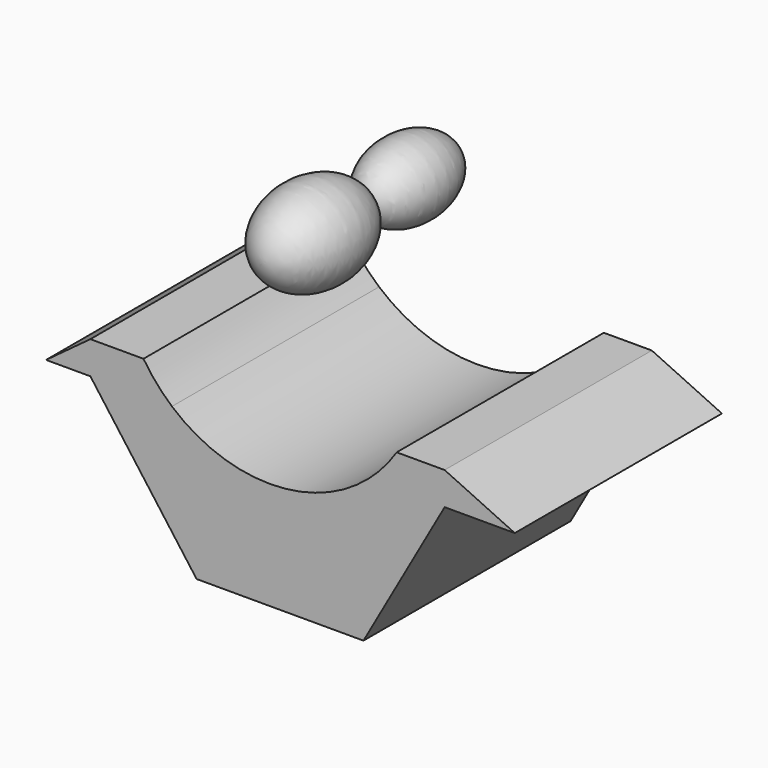
from build123d import *

# Parameters (mm, degrees)
F1_DEPTH = 25.4


# Not quite as in the source:
# - ends of sketch curves that miss each other by under 0.0002 mm in the source are joined


with BuildPart() as f1:
    # F0 (on Front) → F1 (new body)
    with BuildSketch(Plane.XZ):
        with BuildLine():
            Line((-18.7875360372, -14.8434843868), (-26.7906785011, -14.8434843868))
            Line((-26.7906785011, -14.8434843868), (-16.3692074327, -28.9628971368))
            Line((-16.3692074327, -28.9628971368), (0, -28.9628971368))
            Line((0, -28.9628971368), (7.9647982493, -14.8434843868))
            Line((7.9647982493, -14.8434843868), (0.4659200925, -14.8434843868))
            ThreePointArc((0.4659200925, -14.8434843868), (-9.1608079724, -18.4115854923), (-18.7875360372, -14.8434843868))
        make_face()
        with BuildLine():
            Line((-31.1351139098, -14.8434843868), (-26.7906785011, -14.8434843868))
            Line((-26.7906785011, -14.8434843868), (-18.7875360372, -14.8434843868))
            ThreePointArc((-18.7875360372, -14.8434843868), (-20.2997307946, -13.3411894824), (-21.5799429669, -11.6368773754))
            Line((-21.5799429669, -11.6368773754), (-26.7906785011, -11.6368773754))
            Line((-26.7906785011, -11.6368773754), (-31.1351139098, -14.8434843868))
        make_face()
        with BuildLine():
            ThreePointArc((3.2583270222, -11.6368773754), (1.9781148499, -13.3411894824), (0.4659200925, -14.8434843868))
            Line((0.4659200925, -14.8434843868), (7.9647982493, -14.8434843868))
            Line((7.9647982493, -14.8434843868), (14.8434843868, -14.8434843868))
            Line((14.8434843868, -14.8434843868), (7.9647982493, -11.6368773754))
            Line((7.9647982493, -11.6368773754), (3.2583270222, -11.6368773754))
        make_face()
    extrude(amount=F1_DEPTH)


with BuildPart() as f3:
    # F2 (on Top) → F3 (revolve)
    with BuildSketch(Plane.XY):
        with BuildLine():
            Line((-10.4990489781, -12.3092317954), (-10.4990489781, -1.4481449034))
            add(Edge.make_bspline(
                [(-10.4990489781, -1.4481449034), (-14.1520259814, -1.4481449034), (-14.1520259814, -6.8786880001), (-14.1520259814, -12.3092310969), (-10.4990489781, -12.3092317954)],
                knots=[0, 0, 0, 1.5707963268, 1.5707963268, 3.1415926536, 3.1415926536, 3.1415926536], degree=2, weights=[1, 0.7071067812, 1, 0.7071067812, 1]))
        make_face()
    revolve(axis=Axis((-10.4990489781, -13.0333028501, 0), (0, -1, 0)))


with BuildPart() as f3b:
    # F2 (on Top) → F3, piece 2 (revolve)
    with BuildSketch(Plane.XY):
        with BuildLine():
            add(Edge.make_bspline(
                [(-10.4990489781, -24.6184607968), (-6.0316230931, -24.6184607968), (-6.0316230931, -18.4638462961), (-6.0316230931, -12.3092317954), (-10.4990489781, -12.3092317954)],
                knots=[3.1415926536, 3.1415926536, 3.1415926536, 4.7123889804, 4.7123889804, 6.2831853072, 6.2831853072, 6.2831853072], degree=2, weights=[1, 0.7071067812, 1, 0.7071067812, 1]))
            Line((-10.4990489781, -12.3092317954), (-10.4990489781, -24.6184607968))
        make_face()
    revolve(axis=Axis((-10.4990489781, -13.0333028501, 0), (0, -1, 0)))


solid = Compound([f1.part, f3.part, f3b.part])
